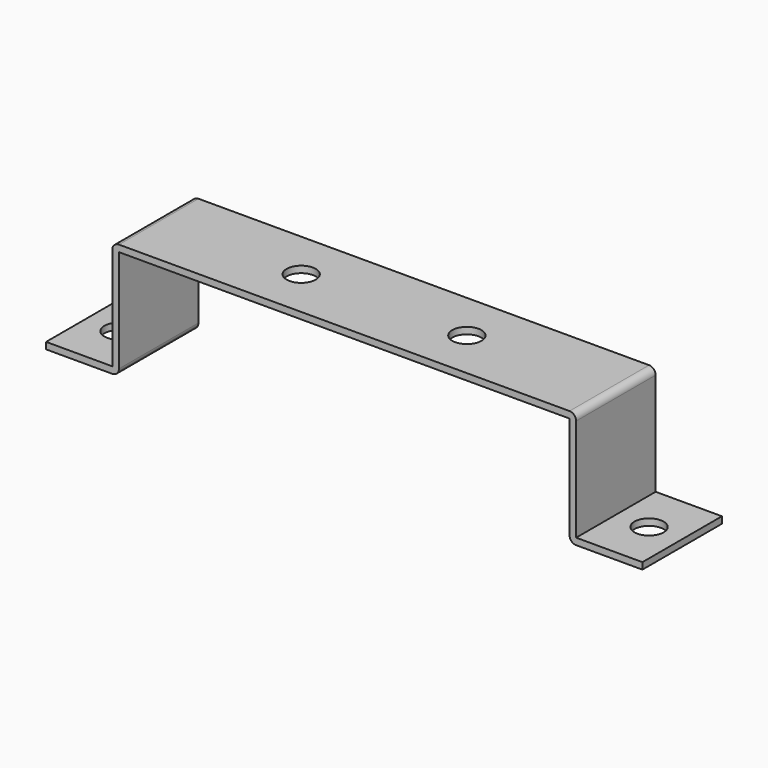
from build123d import *

# Parameters (mm, degrees)
F1_DEPTH = 30
F2_R     = 4.4
F3_R     = 4.4
F4_DEPTH = 25
F5_R     = 2
F6_R     = 2


# Not quite as in the source:
# - a feature names something its author has since deleted; it is built from what else it names


with BuildPart() as f1:
    # F0 (on Front) → F1 (new body)
    with BuildSketch(Plane.XZ):
        Polygon((90, -1), (90, 1), (70, 1), (70, 34), (-70, 34), (-70, 1), (-90, 1), (-90, -1), (-68, -1), (-68, 32), (68, 32), (68, -1), align=None)
    extrude(amount=F1_DEPTH)

    # F2 (on face) + F3 (on face) → F4 (cut)
    with BuildSketch(Plane.XY.offset(1)):
        with Locations((-80, -15)):
            Circle(F2_R)
        with Locations((80, -15)):
            Circle(F2_R)
    with BuildSketch(Plane.XY.offset(34)):
        with Locations((-25, -15)):
            Circle(F3_R)
        with Locations((25, -15)):
            Circle(F3_R)
    extrude(amount=-F4_DEPTH, mode=Mode.SUBTRACT)

    # F5
    f5_edges = [f1.edges().sort_by_distance(p)[0] for p in [
        (-70, -15, 34),
        (70, -15, 34),
    ]]
    fillet(f5_edges, radius=F5_R)

    # F6
    f6_edges = [f1.edges().sort_by_distance(p)[0] for p in [
        (68, -15, -1),
        (-68, -15, -1),
    ]]
    fillet(f6_edges, radius=F6_R)


solid = f1.part
